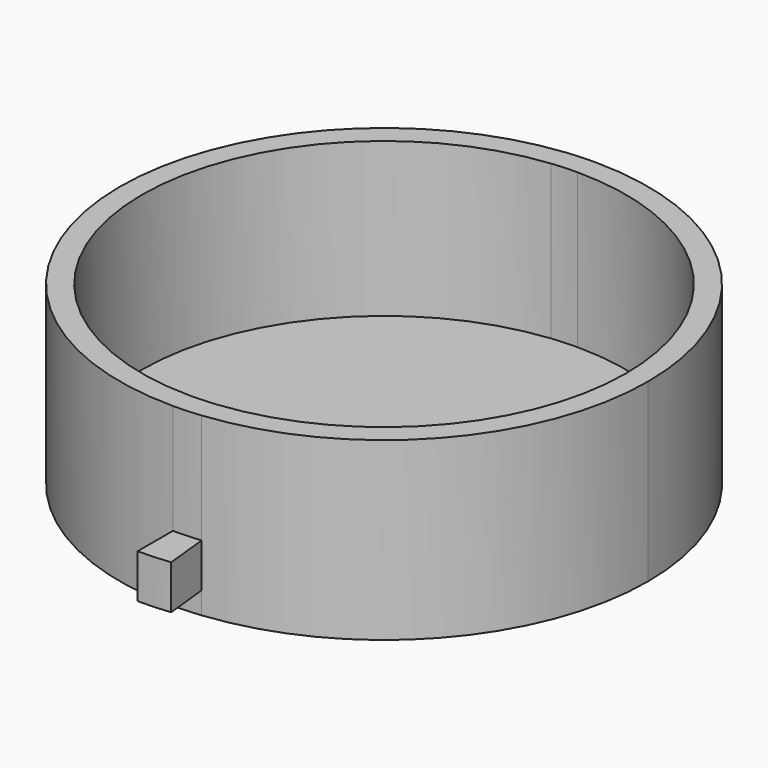
from build123d import *
from build123d import SkipClean  # not in build123d's __all__

# Parameters (mm, degrees)
F1_DEPTH = 50.8
F2_DEPTH = 19.05
F3_DEPTH = 6.35
F4_DEPTH = 6.35


# Not quite as in the source:
# - after a boolean that leaves OpenCascade's solid faulty, fix() repairs it


with BuildPart() as f1:
    # F0 (on Top) → F1 (new body)
    with BuildSketch(Plane.XY):
        with BuildLine():
            Line((-7.3013131592, 69.4673543915), (-7.965068901, 75.7825684271))
            ThreePointArc((-7.965068901, 75.7825684271), (-76.0955705483, -3.9879998657), (0, -76.2))
            Line((0, -76.2), (0, -69.85))
            ThreePointArc((0, -69.85), (-69.7542730026, -3.6556665436), (-7.3013131592, 69.4673543915))
        make_face()
        with BuildLine():
            Line((0, 69.85), (0, 76.2))
            ThreePointArc((0, 76.2), (-3.9879998657, 76.0955705483), (-7.965068901, 75.7825684271))
            Line((-7.965068901, 75.7825684271), (-7.3013131592, 69.4673543915))
            ThreePointArc((-7.3013131592, 69.4673543915), (-3.6556665436, 69.7542730026), (0, 69.85))
        make_face()
        with BuildLine():
            ThreePointArc((0, -76.2), (3.9879998657, -76.0955705483), (7.965068901, -75.7825684271))
            Line((7.965068901, -75.7825684271), (7.3013131592, -69.4673543915))
            ThreePointArc((7.3013131592, -69.4673543915), (3.6556665436, -69.7542730026), (0, -69.85))
            Line((0, -69.85), (0, -76.2))
        make_face()
        with BuildLine():
            ThreePointArc((7.965068901, -75.7825684271), (56.6276357014, -50.9877522045), (76.2, 0))
            ThreePointArc((76.2, 0), (53.8815367264, 53.8815367264), (0, 76.2))
            Line((0, 76.2), (0, 69.85))
            ThreePointArc((0, 69.85), (49.3914086659, 49.3914086659), (69.85, 0))
            ThreePointArc((69.85, 0), (51.9086660596, -46.7387728542), (7.3013131592, -69.4673543915))
            Line((7.3013131592, -69.4673543915), (7.965068901, -75.7825684271))
        make_face()
    extrude(amount=F1_DEPTH)

    # F0 (on Top) → F2 (join)
    with BuildSketch(Plane.XY):
        with BuildLine():
            ThreePointArc((-7.965068901, 75.7825684271), (-3.9879998657, 76.0955705483), (0, 76.2))
            Line((0, 76.2), (0, 88.9))
            ThreePointArc((0, 88.9), (-4.65266651, 88.7781656397), (-9.2925803845, 88.4129964982))
            Line((-9.2925803845, 88.4129964982), (-7.965068901, 75.7825684271))
        make_face()
        with BuildLine():
            Line((9.2925803845, -88.4129964982), (7.965068901, -75.7825684271))
            ThreePointArc((7.965068901, -75.7825684271), (3.9879998657, -76.0955705483), (0, -76.2))
            Line((0, -76.2), (0, -88.9))
            ThreePointArc((0, -88.9), (4.65266651, -88.7781656397), (9.2925803845, -88.4129964982))
        make_face()
    extrude(amount=F2_DEPTH)

    # F0 (on Top) → F3 (cut)
    with BuildSketch(Plane.XY):
        with BuildLine():
            Line((9.2925803845, -88.4129964982), (7.965068901, -75.7825684271))
            ThreePointArc((7.965068901, -75.7825684271), (3.9879998657, -76.0955705483), (0, -76.2))
            Line((0, -76.2), (0, -88.9))
            ThreePointArc((0, -88.9), (4.65266651, -88.7781656397), (9.2925803845, -88.4129964982))
        make_face()
        with BuildLine():
            ThreePointArc((-7.965068901, 75.7825684271), (-3.9879998657, 76.0955705483), (0, 76.2))
            Line((0, 76.2), (0, 88.9))
            ThreePointArc((0, 88.9), (-4.65266651, 88.7781656397), (-9.2925803845, 88.4129964982))
            Line((-9.2925803845, 88.4129964982), (-7.965068901, 75.7825684271))
        make_face()
    with SkipClean():  # cleaning this boolean's faces spoils the solid; the shape is the same uncleaned
        extrude(amount=F3_DEPTH, mode=Mode.SUBTRACT)

    # F0 (on Top) → F4 (join)
    with BuildSketch(Plane.XY):
        with BuildLine():
            Line((0, 0), (-7.3013131592, 69.4673543915))
            ThreePointArc((-7.3013131592, 69.4673543915), (-69.7542730026, -3.6556665436), (0, -69.85))
            Line((0, -69.85), (0, 0))
        make_face()
        with BuildLine():
            Line((0, 0), (0, 69.85))
            ThreePointArc((0, 69.85), (-3.6556665436, 69.7542730026), (-7.3013131592, 69.4673543915))
            Line((-7.3013131592, 69.4673543915), (0, 0))
        make_face()
        with BuildLine():
            ThreePointArc((69.85, 0), (49.3914086659, 49.3914086659), (0, 69.85))
            Line((0, 69.85), (0, 0))
            Line((0, 0), (7.3013131592, -69.4673543915))
            ThreePointArc((7.3013131592, -69.4673543915), (51.9086660596, -46.7387728542), (69.85, 0))
        make_face()
        with BuildLine():
            ThreePointArc((0, -69.85), (3.6556665436, -69.7542730026), (7.3013131592, -69.4673543915))
            Line((7.3013131592, -69.4673543915), (0, 0))
            Line((0, 0), (0, -69.85))
        make_face()
    extrude(amount=F4_DEPTH)

    add(f1.part.fix(), mode=Mode.REPLACE)


solid = f1.part
